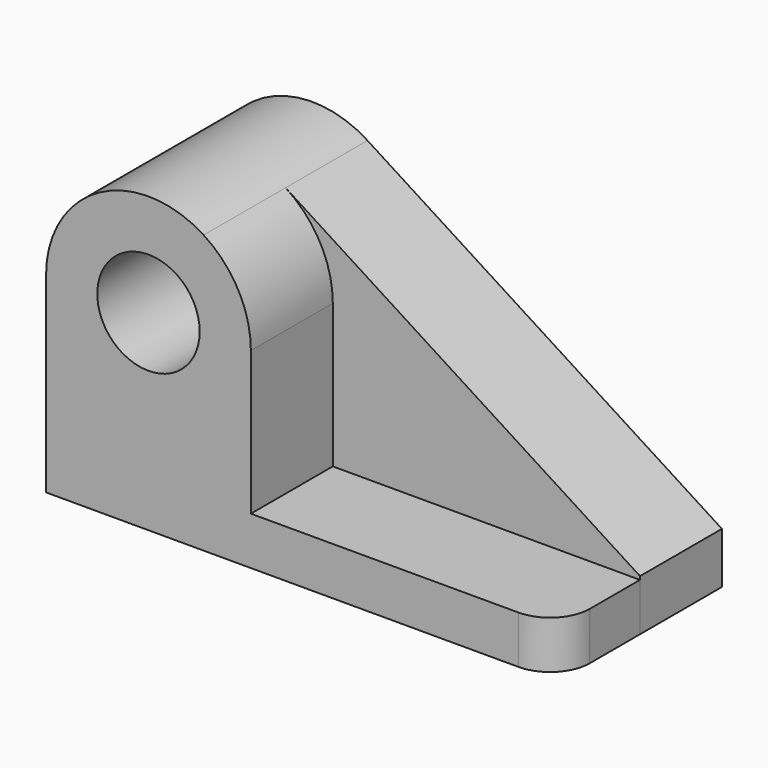
from build123d import *
from build123d import SkipClean  # not in build123d's __all__

# Parameters (mm, degrees)
F1_DEPTH = 25.4
F2_R     = 12.7
F3_DEPTH = 25.4
F4_R     = 9.8113639175


with BuildPart() as f1:
    # F0 (on Front) → F1 (new body)
    with BuildSketch(Plane.XZ):
        with BuildLine():
            ThreePointArc((-37.8463725496, 72.1998437426), (-63.7276630417, 73.0788204047), (-76.9287220478, 50.8))
            Line((-76.9287220478, 50.8), (-76.9287220478, 3.2882173546))
            Line((-76.9287220478, 3.2882173546), (50.0712779522, 3.2882173546))
            Line((50.0712779522, 3.2882173546), (50.0712779522, 15.9882173546))
            Line((50.0712779522, 15.9882173546), (-37.8463725496, 72.1998437426))
        make_face()
        with BuildLine():
            ThreePointArc((-64.2287220478, 50.8), (-51.5287220478, 63.5), (-38.8287220478, 50.8))
            ThreePointArc((-38.8287220478, 50.8), (-51.5287220478, 38.1), (-64.2287220478, 50.8))
        make_face(mode=Mode.SUBTRACT)
    extrude(amount=F1_DEPTH)

    # F2 (on face) → F3 (join)
    with BuildSketch(Plane.XZ.offset(25.4)):
        with BuildLine():
            Line((-26.1287220478, 15.9882173546), (-26.1287220478, 50.8))
            ThreePointArc((-26.1287220478, 50.8), (-29.2499016431, 62.9989409939), (-37.8463725496, 72.1998437426))
            ThreePointArc((-37.8463725496, 72.1998437426), (-63.7276630417, 73.0788204047), (-76.9287220478, 50.8))
            Line((-76.9287220478, 50.8), (-76.9287220478, 15.1695013046))
            Line((-76.9287220478, 15.1695013046), (-76.9287220478, 3.2882173546))
            Line((-76.9287220478, 3.2882173546), (50.0712779522, 3.2882173546))
            Line((50.0712779522, 3.2882173546), (50.0712779522, 15.1695013046))
            Line((50.0712779522, 15.1695013046), (-26.1287220478, 15.1695013046))
            Line((-26.1287220478, 15.1695013046), (-26.1287220478, 15.9882173546))
        make_face()
        with Locations((-51.5287220478, 50.8)):
            Circle(F2_R, mode=Mode.SUBTRACT)
    with SkipClean():  # cleaning this boolean's faces spoils the solid; the shape is the same uncleaned
        extrude(amount=F3_DEPTH)

    # F4
    f4_edges = [f1.edges().sort_by_distance(p)[0] for p in [
        (50.071278, -50.8, 9.228859),
    ]]
    fillet(f4_edges, radius=F4_R)


solid = f1.part
